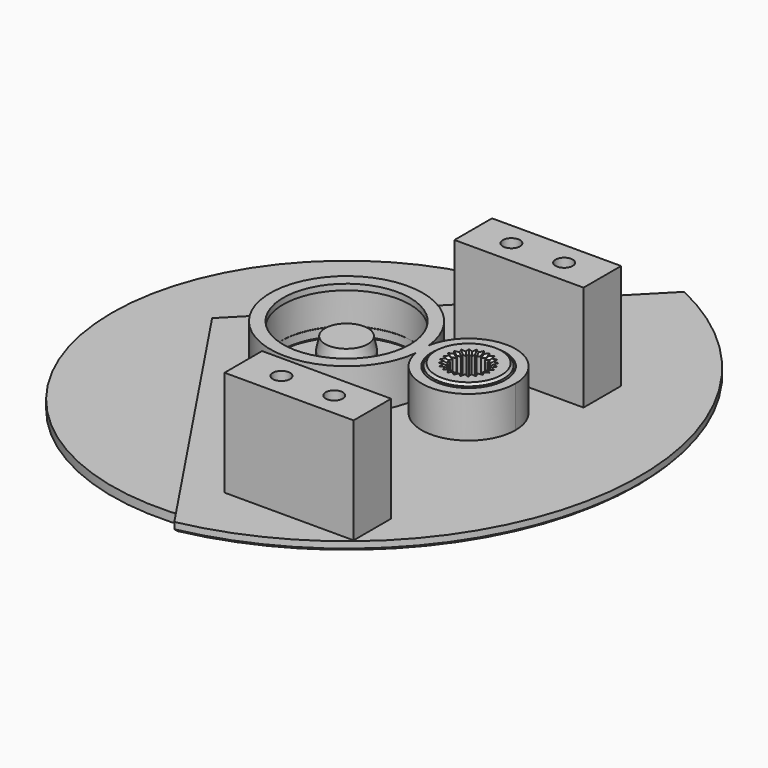
from build123d import *

# Parameters (mm, degrees)
F0_R           = 40
F1_DEPTH       = 1.5
F3_DEPTH       = 3
F4_R           = 4.05
F5_DEPTH       = 6.5
F6_SIZE2       = 2
F6_SIZE        = 0.4
F8_R           = 2
F9_DEPTH       = 2.6
F10_R          = 6
F11_DEPTH      = 9
F12_R          = 11.3
F12_R_2        = 6.2
F13_DEPTH      = 1.5
F14_SIZE       = 0.4
F15_R          = 6.3
F15_R_2        = 11.2
F16_DEPTH      = 7
F17_R          = 11.2
F17_R_2        = 10.8
F18_DEPTH      = 1
F19_C1_SIZE    = 0.4
F19_C2_SIZE    = 0.4
F19_C3_SIZE    = 0.4
F19_C4_SIZE    = 0.4
F19_C5_SIZE    = 0.4
F19_C6_SIZE    = 0.4
F19_C7_SIZE    = 0.4
F19_C8_SIZE    = 0.4
F19_C9_SIZE    = 0.4
F19_C10_SIZE   = 0.4
F19_C11_SIZE   = 0.4
F19_C12_SIZE   = 0.4
F19_C13_SIZE   = 0.4
F19_C14_SIZE   = 0.4
F19_C15_SIZE   = 0.4
F19_C16_SIZE   = 0.4
F19_C17_SIZE   = 0.4
F19_C18_SIZE   = 0.4
F19_C19_SIZE   = 0.4
F19_C20_SIZE   = 0.4
F19_C21_SIZE   = 0.4
F19_C22_SIZE   = 0.4
F19_C23_SIZE   = 0.4
F19_C24_SIZE   = 0.4
F19_C25_SIZE   = 0.4
F19_C26_SIZE   = 0.4
F19_C27_SIZE   = 0.4
F19_C28_SIZE   = 0.4
F19_C29_SIZE   = 0.4
F19_C30_SIZE   = 0.4
F19_C31_SIZE   = 0.4
F19_C32_SIZE   = 0.4
F19_C33_SIZE   = 0.4
F19_C34_SIZE   = 0.4
F19_C35_SIZE   = 0.4
F19_C36_SIZE   = 0.4
F19_C37_SIZE   = 0.4
F19_C38_SIZE   = 0.4
F19_C39_SIZE   = 0.4
F19_C40_SIZE   = 0.4
F19_C41_SIZE   = 0.4
F19_C42_SIZE   = 0.4
F19_C43_SIZE   = 0.4
F19_C44_SIZE   = 0.4
F19_C45_SIZE   = 0.4
F19_C46_SIZE   = 0.4
F19_C47_SIZE   = 0.4
F19_C48_SIZE   = 0.4
F19_C49_SIZE   = 0.4
F19_2_S5_R     = 11.3
F19_2_T6_DEPTH = 18
F21_W          = 22
F21_H          = 8
F21_R          = 1.4665195189
F22_DEPTH      = 18


# Not quite as in the source:
# - a fillet or chamfer that OpenCascade refuses, or shapes differently, is made with other operations: its cross-section is extruded or revolved along the edge and cut away or added


with BuildPart() as f1:
    # F0 (on Top) → F1 (new body)
    with BuildSketch(Plane.XY):
        Circle(F0_R)
    extrude(amount=F1_DEPTH)

    # F2 (on face) → F3 (join)
    with BuildSketch(Plane.XY.offset(1.5)):
        with BuildLine():
            ThreePointArc((6.1294095226, -0.4829629131), (6.3966766701, -0.3043807145), (6.5, 0))
            ThreePointArc((6.5, 0), (6.3966766701, 0.3043807145), (6.1294095226, 0.4829629131))
            ThreePointArc((6.1294095226, 0.4829629131), (5.5, 0), (6.1294095226, -0.4829629131))
        make_face()
        with BuildLine():
            ThreePointArc((6.1294095226, -0.4829629131), (5.5, 0), (6.1294095226, 0.4829629131))
            Line((6.1294095226, 0.4829629131), (4.19755787, 1.0006010033))
            Line((4.19755787, 1.0006010033), (4.1590994684, 1.1144273438))
            Line((4.1590994684, 1.1144273438), (4.1354922509, 1.232233047))
            Line((4.1354922509, 1.232233047), (5.5497058133, 2.6464466094))
            ThreePointArc((5.5497058133, 2.6464466094), (4.7631397208, 2.75), (5.0667429002, 3.4829629131))
            Line((5.0667429002, 3.4829629131), (3.1348912476, 2.9653248229))
            Line((3.1348912476, 2.9653248229), (3.0446721246, 3.0446721246))
            Line((3.0446721246, 3.0446721246), (2.9653248229, 3.1348912476))
            Line((2.9653248229, 3.1348912476), (3.4829629131, 5.0667429002))
            ThreePointArc((3.4829629131, 5.0667429002), (2.75, 4.7631397208), (2.6464466094, 5.5497058133))
            Line((2.6464466094, 5.5497058133), (1.232233047, 4.1354922509))
            Line((1.232233047, 4.1354922509), (1.1144273438, 4.1590994684))
            Line((1.1144273438, 4.1590994684), (1.0006010033, 4.19755787))
            Line((1.0006010033, 4.19755787), (0.4829629131, 6.1294095226))
            ThreePointArc((0.4829629131, 6.1294095226), (0.4957224307, 6.0652630961), (0.5, 6))
            ThreePointArc((0.5, 6), (-0.0652630961, 5.5042775693), (-0.4829629131, 6.1294095226))
            Line((-0.4829629131, 6.1294095226), (-1.0006010033, 4.19755787))
            Line((-1.0006010033, 4.19755787), (-1.1144273438, 4.1590994684))
            Line((-1.1144273438, 4.1590994684), (-1.232233047, 4.1354922509))
            Line((-1.232233047, 4.1354922509), (-2.6464466094, 5.5497058133))
            ThreePointArc((-2.6464466094, 5.5497058133), (-2.5380602337, 5.3874941389), (-2.5, 5.1961524227))
            ThreePointArc((-2.5, 5.1961524227), (-2.9347369039, 4.700429992), (-3.4829629131, 5.0667429002))
            Line((-3.4829629131, 5.0667429002), (-2.9653248229, 3.1348912476))
            Line((-2.9653248229, 3.1348912476), (-3.0446721246, 3.0446721246))
            Line((-3.0446721246, 3.0446721246), (-3.1348912476, 2.9653248229))
            Line((-3.1348912476, 2.9653248229), (-5.0667429002, 3.4829629131))
            ThreePointArc((-5.0667429002, 3.4829629131), (-4.7994757526, 3.3043807145), (-4.6961524227, 3))
            ThreePointArc((-4.6961524227, 3), (-5.0048107065, 2.5380602337), (-5.5497058133, 2.6464466094))
            Line((-5.5497058133, 2.6464466094), (-4.1354922509, 1.232233047))
            Line((-4.1354922509, 1.232233047), (-4.1590994684, 1.1144273438))
            Line((-4.1590994684, 1.1144273438), (-4.19755787, 1.0006010033))
            Line((-4.19755787, 1.0006010033), (-6.1294095226, 0.4829629131))
            ThreePointArc((-6.1294095226, 0.4829629131), (-5.6956192855, 0.3966766701), (-5.5, 0))
            ThreePointArc((-5.5, 0), (-5.6956192855, -0.3966766701), (-6.1294095226, -0.4829629131))
            Line((-6.1294095226, -0.4829629131), (-4.19755787, -1.0006010033))
            Line((-4.19755787, -1.0006010033), (-4.1590994684, -1.1144273438))
            Line((-4.1590994684, -1.1144273438), (-4.1354922509, -1.232233047))
            Line((-4.1354922509, -1.232233047), (-5.5497058133, -2.6464466094))
            ThreePointArc((-5.5497058133, -2.6464466094), (-5.0048107065, -2.5380602337), (-4.6961524227, -3))
            ThreePointArc((-4.6961524227, -3), (-4.7994757526, -3.3043807145), (-5.0667429002, -3.4829629131))
            Line((-5.0667429002, -3.4829629131), (-3.1348912476, -2.9653248229))
            Line((-3.1348912476, -2.9653248229), (-3.0446721246, -3.0446721246))
            Line((-3.0446721246, -3.0446721246), (-2.9653248229, -3.1348912476))
            Line((-2.9653248229, -3.1348912476), (-3.4829629131, -5.0667429002))
            ThreePointArc((-3.4829629131, -5.0667429002), (-2.9347369039, -4.700429992), (-2.5, -5.1961524227))
            ThreePointArc((-2.5, -5.1961524227), (-2.5380602337, -5.3874941389), (-2.6464466094, -5.5497058133))
            Line((-2.6464466094, -5.5497058133), (-1.232233047, -4.1354922509))
            Line((-1.232233047, -4.1354922509), (-1.1144273438, -4.1590994684))
            Line((-1.1144273438, -4.1590994684), (-1.0006010033, -4.19755787))
            Line((-1.0006010033, -4.19755787), (-0.4829629131, -6.1294095226))
            ThreePointArc((-0.4829629131, -6.1294095226), (-0.0652630961, -5.5042775693), (0.5, -6))
            ThreePointArc((0.5, -6), (0.4957224307, -6.0652630961), (0.4829629131, -6.1294095226))
            Line((0.4829629131, -6.1294095226), (1.0006010033, -4.19755787))
            Line((1.0006010033, -4.19755787), (1.1144273438, -4.1590994684))
            Line((1.1144273438, -4.1590994684), (1.232233047, -4.1354922509))
            Line((1.232233047, -4.1354922509), (2.6464466094, -5.5497058133))
            ThreePointArc((2.6464466094, -5.5497058133), (2.75, -4.7631397208), (3.4829629131, -5.0667429002))
            Line((3.4829629131, -5.0667429002), (2.9653248229, -3.1348912476))
            Line((2.9653248229, -3.1348912476), (3.0446721246, -3.0446721246))
            Line((3.0446721246, -3.0446721246), (3.1348912476, -2.9653248229))
            Line((3.1348912476, -2.9653248229), (5.0667429002, -3.4829629131))
            ThreePointArc((5.0667429002, -3.4829629131), (4.7631397208, -2.75), (5.5497058133, -2.6464466094))
            Line((5.5497058133, -2.6464466094), (4.1354922509, -1.232233047))
            Line((4.1354922509, -1.232233047), (4.1590994684, -1.1144273438))
            Line((4.1590994684, -1.1144273438), (4.19755787, -1.0006010033))
            Line((4.19755787, -1.0006010033), (6.1294095226, -0.4829629131))
        make_face()
        with BuildLine():
            ThreePointArc((5.0667429002, 3.4829629131), (4.7631397208, 2.75), (5.5497058133, 2.6464466094))
            ThreePointArc((5.5497058133, 2.6464466094), (5.658092189, 2.8086582838), (5.6961524227, 3))
            ThreePointArc((5.6961524227, 3), (5.5005331372, 3.3966766701), (5.0667429002, 3.4829629131))
        make_face()
        with BuildLine():
            ThreePointArc((5.6961524227, -3), (5.658092189, -2.8086582838), (5.5497058133, -2.6464466094))
            ThreePointArc((5.5497058133, -2.6464466094), (4.7631397208, -2.75), (5.0667429002, -3.4829629131))
            ThreePointArc((5.0667429002, -3.4829629131), (5.5005331372, -3.3966766701), (5.6961524227, -3))
        make_face()
        with BuildLine():
            ThreePointArc((2.6464466094, 5.5497058133), (2.75, 4.7631397208), (3.4829629131, 5.0667429002))
            ThreePointArc((3.4829629131, 5.0667429002), (3.4957224307, 5.1308893266), (3.5, 5.1961524227))
            ThreePointArc((3.5, 5.1961524227), (3.1913417162, 5.658092189), (2.6464466094, 5.5497058133))
        make_face()
        with BuildLine():
            ThreePointArc((3.5, -5.1961524227), (3.4957224307, -5.1308893266), (3.4829629131, -5.0667429002))
            ThreePointArc((3.4829629131, -5.0667429002), (2.75, -4.7631397208), (2.6464466094, -5.5497058133))
            ThreePointArc((2.6464466094, -5.5497058133), (3.1913417162, -5.658092189), (3.5, -5.1961524227))
        make_face()
        with BuildLine():
            ThreePointArc((0.5, 6), (0.4957224307, 6.0652630961), (0.4829629131, 6.1294095226))
            ThreePointArc((0.4829629131, 6.1294095226), (0, 6.5), (-0.4829629131, 6.1294095226))
            ThreePointArc((-0.4829629131, 6.1294095226), (-0.0652630961, 5.5042775693), (0.5, 6))
        make_face()
        with BuildLine():
            ThreePointArc((-0.4829629131, -6.1294095226), (0, -6.5), (0.4829629131, -6.1294095226))
            ThreePointArc((0.4829629131, -6.1294095226), (0.4957224307, -6.0652630961), (0.5, -6))
            ThreePointArc((0.5, -6), (-0.0652630961, -5.5042775693), (-0.4829629131, -6.1294095226))
        make_face()
        with BuildLine():
            ThreePointArc((-2.5, 5.1961524227), (-2.5380602337, 5.3874941389), (-2.6464466094, 5.5497058133))
            ThreePointArc((-2.6464466094, 5.5497058133), (-3.25, 5.6291651246), (-3.4829629131, 5.0667429002))
            ThreePointArc((-3.4829629131, 5.0667429002), (-2.9347369039, 4.700429992), (-2.5, 5.1961524227))
        make_face()
        with BuildLine():
            ThreePointArc((-3.4829629131, -5.0667429002), (-3.25, -5.6291651246), (-2.6464466094, -5.5497058133))
            ThreePointArc((-2.6464466094, -5.5497058133), (-2.5380602337, -5.3874941389), (-2.5, -5.1961524227))
            ThreePointArc((-2.5, -5.1961524227), (-2.9347369039, -4.700429992), (-3.4829629131, -5.0667429002))
        make_face()
        with BuildLine():
            ThreePointArc((-4.6961524227, 3), (-4.7994757526, 3.3043807145), (-5.0667429002, 3.4829629131))
            ThreePointArc((-5.0667429002, 3.4829629131), (-5.6291651246, 3.25), (-5.5497058133, 2.6464466094))
            ThreePointArc((-5.5497058133, 2.6464466094), (-5.0048107065, 2.5380602337), (-4.6961524227, 3))
        make_face()
        with BuildLine():
            ThreePointArc((-5.5497058133, -2.6464466094), (-5.6291651246, -3.25), (-5.0667429002, -3.4829629131))
            ThreePointArc((-5.0667429002, -3.4829629131), (-4.7994757526, -3.3043807145), (-4.6961524227, -3))
            ThreePointArc((-4.6961524227, -3), (-5.0048107065, -2.5380602337), (-5.5497058133, -2.6464466094))
        make_face()
        with BuildLine():
            ThreePointArc((-5.5, 0), (-5.6956192855, 0.3966766701), (-6.1294095226, 0.4829629131))
            ThreePointArc((-6.1294095226, 0.4829629131), (-6.5, 0), (-6.1294095226, -0.4829629131))
            ThreePointArc((-6.1294095226, -0.4829629131), (-5.6956192855, -0.3966766701), (-5.5, 0))
        make_face()
    extrude(amount=F3_DEPTH)

    # F4 (on face) → F5 (join)
    with BuildSketch(Plane.XY.offset(4.5)):
        Circle(F4_R)
    extrude(amount=F5_DEPTH)

    # F6
    f6_edges = [f1.edges().sort_by_distance(p)[0] for p in [
        (-4.05, 0, 11),
    ]]
    f6_side = f1.faces().sort_by_distance((0, 0, 11))[0]
    chamfer(f6_edges, length=F6_SIZE, length2=F6_SIZE2, reference=f6_side)


with BuildPart() as f9:
    # F8 (on offset) → F9 (new body)
    with BuildSketch(Plane.XY.offset(4.75)):
        with BuildLine():
            ThreePointArc((36.005212086, -0.5638155725), (36.2914912266, -0.3441458618), (36.4, 0))
            ThreePointArc((36.4, 0), (36.2914912266, 0.3441458618), (36.005212086, 0.5638155725))
            ThreePointArc((36.005212086, 0.5638155725), (35.2, 0), (36.005212086, -0.5638155725))
        make_face()
        with BuildLine():
            ThreePointArc((36.005212086, -0.5638155725), (35.2, 0), (36.005212086, 0.5638155725))
            Line((36.005212086, 0.5638155725), (34.5956731548, 1.0768457875))
            Line((34.5956731548, 1.0768457875), (34.2894922687, 1.7759253484))
            Line((34.2894922687, 1.7759253484), (34.4043051897, 2.5304297954))
            Line((34.4043051897, 2.5304297954), (35.6330332561, 3.39079445))
            ThreePointArc((35.6330332561, 3.39079445), (34.7093318986, 3.7269942495), (35.34118084, 4.4800024954))
            Line((35.34118084, 4.4800024954), (33.8468887928, 4.6107361095))
            Line((33.8468887928, 4.6107361095), (33.3702056631, 5.2067496675))
            Line((33.3702056631, 5.2067496675), (33.2858263081, 5.9652607695))
            Line((33.2858263081, 5.9652607695), (34.2500077226, 7.1143274342))
            ThreePointArc((34.2500077226, 7.1143274342), (33.2707658145, 7.2), (33.6861921502, 8.0908846518))
            Line((33.6861921502, 8.0908846518), (32.2089805206, 7.8304123853))
            Line((32.2089805206, 7.8304123853), (31.5942803147, 8.2827426013))
            Line((31.5942803147, 8.2827426013), (31.3164589974, 8.9935690802))
            Line((31.3164589974, 8.9935690802), (31.95038639, 10.3530307608))
            ThreePointArc((31.95038639, 10.3530307608), (30.9823376491, 10.1823376491), (31.1530307608, 11.15038639))
            Line((31.1530307608, 11.15038639), (29.7935690802, 10.5164589974))
            Line((29.7935690802, 10.5164589974), (29.0827426013, 10.7942803147))
            Line((29.0827426013, 10.7942803147), (28.6304123853, 11.4089805206))
            Line((28.6304123853, 11.4089805206), (28.8908846518, 12.8861921502))
            ThreePointArc((28.8908846518, 12.8861921502), (28, 12.4707658145), (27.9143274342, 13.4500077226))
            Line((27.9143274342, 13.4500077226), (26.7652607695, 12.4858263081))
            Line((26.7652607695, 12.4858263081), (26.0067496675, 12.5702056631))
            Line((26.0067496675, 12.5702056631), (25.4107361095, 13.0468887928))
            Line((25.4107361095, 13.0468887928), (25.2800024954, 14.54118084))
            ThreePointArc((25.2800024954, 14.54118084), (25.2817146095, 14.5150590268), (25.2822856765, 14.4888873943))
            ThreePointArc((25.2822856765, 14.4888873943), (24.5018621968, 13.9166572239), (24.19079445, 14.8330332561))
            Line((24.19079445, 14.8330332561), (23.3304297954, 13.6043051897))
            Line((23.3304297954, 13.6043051897), (22.5759253484, 13.4894922687))
            Line((22.5759253484, 13.4894922687), (21.8768457875, 13.7956731548))
            Line((21.8768457875, 13.7956731548), (21.3638155725, 15.205212086))
            ThreePointArc((21.3638155725, 15.205212086), (21.3908846518, 15.1041889066), (21.4, 15))
            ThreePointArc((21.4, 15), (20.6958110934, 14.4091153482), (20.2361844275, 15.205212086))
            Line((20.2361844275, 15.205212086), (19.7231542125, 13.7956731548))
            Line((19.7231542125, 13.7956731548), (19.0240746516, 13.4894922687))
            Line((19.0240746516, 13.4894922687), (18.2695702046, 13.6043051897))
            Line((18.2695702046, 13.6043051897), (17.40920555, 14.8330332561))
            ThreePointArc((17.40920555, 14.8330332561), (17.4899444939, 14.669310874), (17.5177143235, 14.4888873943))
            ThreePointArc((17.5177143235, 14.4888873943), (16.891542691, 13.8894584614), (16.3199975046, 14.54118084))
            Line((16.3199975046, 14.54118084), (16.1892638905, 13.0468887928))
            Line((16.1892638905, 13.0468887928), (15.5932503325, 12.5702056631))
            Line((15.5932503325, 12.5702056631), (14.8347392305, 12.4858263081))
            Line((14.8347392305, 12.4858263081), (13.6856725658, 13.4500077226))
            ThreePointArc((13.6856725658, 13.4500077226), (13.8437846722, 13.2439520138), (13.9, 12.9903810568))
            ThreePointArc((13.9, 12.9903810568), (13.3522934456, 12.3926642379), (12.7091153482, 12.8861921502))
            Line((12.7091153482, 12.8861921502), (12.9695876147, 11.4089805206))
            Line((12.9695876147, 11.4089805206), (12.5172573987, 10.7942803147))
            Line((12.5172573987, 10.7942803147), (11.8064309198, 10.5164589974))
            Line((11.8064309198, 10.5164589974), (10.4469692392, 11.15038639))
            ThreePointArc((10.4469692392, 11.15038639), (10.6994331497, 10.9289814828), (10.7933982822, 10.6066017178))
            ThreePointArc((10.7933982822, 10.6066017178), (10.3232620506, 10.0208241135), (9.64961361, 10.3530307608))
            Line((9.64961361, 10.3530307608), (10.2835410026, 8.9935690802))
            Line((10.2835410026, 8.9935690802), (10.0057196853, 8.2827426013))
            Line((10.0057196853, 8.2827426013), (9.3910194794, 7.8304123853))
            Line((9.3910194794, 7.8304123853), (7.9138078498, 8.0908846518))
            ThreePointArc((7.9138078498, 8.0908846518), (8.2692456091, 7.8856725658), (8.4096189432, 7.5))
            ThreePointArc((8.4096189432, 7.5), (8.0148310292, 6.9361844275), (7.3499922774, 7.1143274342))
            Line((7.3499922774, 7.1143274342), (8.3141736919, 5.9652607695))
            Line((8.3141736919, 5.9652607695), (8.2297943369, 5.2067496675))
            Line((8.2297943369, 5.2067496675), (7.7531112072, 4.6107361095))
            Line((7.7531112072, 4.6107361095), (6.25881916, 4.4800024954))
            ThreePointArc((6.25881916, 4.4800024954), (6.7164667302, 4.3246520786), (6.9111126057, 3.8822856765))
            ThreePointArc((6.9111126057, 3.8822856765), (6.5881617736, 3.3500791766), (5.9669667439, 3.39079445))
            Line((5.9669667439, 3.39079445), (7.1956948103, 2.5304297954))
            Line((7.1956948103, 2.5304297954), (7.3105077313, 1.7759253484))
            Line((7.3105077313, 1.7759253484), (7.0043268452, 1.0768457875))
            Line((7.0043268452, 1.0768457875), (5.594787914, 0.5638155725))
            ThreePointArc((5.594787914, 0.5638155725), (6.1441458618, 0.4914912266), (6.4, 0))
            ThreePointArc((6.4, 0), (6.1441458618, -0.4914912266), (5.594787914, -0.5638155725))
            Line((5.594787914, -0.5638155725), (7.0043268452, -1.0768457875))
            Line((7.0043268452, -1.0768457875), (7.3105077313, -1.7759253484))
            Line((7.3105077313, -1.7759253484), (7.1956948103, -2.5304297954))
            Line((7.1956948103, -2.5304297954), (5.9669667439, -3.39079445))
            ThreePointArc((5.9669667439, -3.39079445), (6.5881617736, -3.3500791766), (6.9111126057, -3.8822856765))
            ThreePointArc((6.9111126057, -3.8822856765), (6.7164667302, -4.3246520786), (6.25881916, -4.4800024954))
            Line((6.25881916, -4.4800024954), (7.7531112072, -4.6107361095))
            Line((7.7531112072, -4.6107361095), (8.2297943369, -5.2067496675))
            Line((8.2297943369, -5.2067496675), (8.3141736919, -5.9652607695))
            Line((8.3141736919, -5.9652607695), (7.3499922774, -7.1143274342))
            ThreePointArc((7.3499922774, -7.1143274342), (8.0148310292, -6.9361844275), (8.4096189432, -7.5))
            ThreePointArc((8.4096189432, -7.5), (8.2692456091, -7.8856725658), (7.9138078498, -8.0908846518))
            Line((7.9138078498, -8.0908846518), (9.3910194794, -7.8304123853))
            Line((9.3910194794, -7.8304123853), (10.0057196853, -8.2827426013))
            Line((10.0057196853, -8.2827426013), (10.2835410026, -8.9935690802))
            Line((10.2835410026, -8.9935690802), (9.64961361, -10.3530307608))
            ThreePointArc((9.64961361, -10.3530307608), (10.3232620506, -10.0208241135), (10.7933982822, -10.6066017178))
            ThreePointArc((10.7933982822, -10.6066017178), (10.6994331497, -10.9289814828), (10.4469692392, -11.15038639))
            Line((10.4469692392, -11.15038639), (11.8064309198, -10.5164589974))
            Line((11.8064309198, -10.5164589974), (12.5172573987, -10.7942803147))
            Line((12.5172573987, -10.7942803147), (12.9695876147, -11.4089805206))
            Line((12.9695876147, -11.4089805206), (12.7091153482, -12.8861921502))
            ThreePointArc((12.7091153482, -12.8861921502), (13.3522934456, -12.3926642379), (13.9, -12.9903810568))
            ThreePointArc((13.9, -12.9903810568), (13.8437846722, -13.2439520138), (13.6856725658, -13.4500077226))
            Line((13.6856725658, -13.4500077226), (14.8347392305, -12.4858263081))
            Line((14.8347392305, -12.4858263081), (15.5932503325, -12.5702056631))
            Line((15.5932503325, -12.5702056631), (16.1892638905, -13.0468887928))
            Line((16.1892638905, -13.0468887928), (16.3199975046, -14.54118084))
            ThreePointArc((16.3199975046, -14.54118084), (16.891542691, -13.8894584614), (17.5177143235, -14.4888873943))
            ThreePointArc((17.5177143235, -14.4888873943), (17.4899444939, -14.669310874), (17.40920555, -14.8330332561))
            Line((17.40920555, -14.8330332561), (18.2695702046, -13.6043051897))
            Line((18.2695702046, -13.6043051897), (19.0240746516, -13.4894922687))
            Line((19.0240746516, -13.4894922687), (19.7231542125, -13.7956731548))
            Line((19.7231542125, -13.7956731548), (20.2361844275, -15.205212086))
            ThreePointArc((20.2361844275, -15.205212086), (20.6958110934, -14.4091153482), (21.4, -15))
            ThreePointArc((21.4, -15), (21.3908846518, -15.1041889066), (21.3638155725, -15.205212086))
            Line((21.3638155725, -15.205212086), (21.8768457875, -13.7956731548))
            Line((21.8768457875, -13.7956731548), (22.5759253484, -13.4894922687))
            Line((22.5759253484, -13.4894922687), (23.3304297954, -13.6043051897))
            Line((23.3304297954, -13.6043051897), (24.19079445, -14.8330332561))
            ThreePointArc((24.19079445, -14.8330332561), (24.5018621968, -13.9166572239), (25.2822856765, -14.4888873943))
            ThreePointArc((25.2822856765, -14.4888873943), (25.2817146095, -14.5150590268), (25.2800024954, -14.54118084))
            Line((25.2800024954, -14.54118084), (25.4107361095, -13.0468887928))
            Line((25.4107361095, -13.0468887928), (26.0067496675, -12.5702056631))
            Line((26.0067496675, -12.5702056631), (26.7652607695, -12.4858263081))
            Line((26.7652607695, -12.4858263081), (27.9143274342, -13.4500077226))
            ThreePointArc((27.9143274342, -13.4500077226), (28, -12.4707658145), (28.8908846518, -12.8861921502))
            Line((28.8908846518, -12.8861921502), (28.6304123853, -11.4089805206))
            Line((28.6304123853, -11.4089805206), (29.0827426013, -10.7942803147))
            Line((29.0827426013, -10.7942803147), (29.7935690802, -10.5164589974))
            Line((29.7935690802, -10.5164589974), (31.1530307608, -11.15038639))
            ThreePointArc((31.1530307608, -11.15038639), (30.9823376491, -10.1823376491), (31.95038639, -10.3530307608))
            Line((31.95038639, -10.3530307608), (31.3164589974, -8.9935690802))
            Line((31.3164589974, -8.9935690802), (31.5942803147, -8.2827426013))
            Line((31.5942803147, -8.2827426013), (32.2089805206, -7.8304123853))
            Line((32.2089805206, -7.8304123853), (33.6861921502, -8.0908846518))
            ThreePointArc((33.6861921502, -8.0908846518), (33.2707658145, -7.2), (34.2500077226, -7.1143274342))
            Line((34.2500077226, -7.1143274342), (33.2858263081, -5.9652607695))
            Line((33.2858263081, -5.9652607695), (33.3702056631, -5.2067496675))
            Line((33.3702056631, -5.2067496675), (33.8468887928, -4.6107361095))
            Line((33.8468887928, -4.6107361095), (35.34118084, -4.4800024954))
            ThreePointArc((35.34118084, -4.4800024954), (34.7093318986, -3.7269942495), (35.6330332561, -3.39079445))
            Line((35.6330332561, -3.39079445), (34.4043051897, -2.5304297954))
            Line((34.4043051897, -2.5304297954), (34.2894922687, -1.7759253484))
            Line((34.2894922687, -1.7759253484), (34.5956731548, -1.0768457875))
            Line((34.5956731548, -1.0768457875), (36.005212086, -0.5638155725))
        make_face()
        with Locations((20.8, 0)):
            Circle(F8_R, mode=Mode.SUBTRACT)
        with BuildLine():
            ThreePointArc((35.34118084, 4.4800024954), (34.7093318986, 3.7269942495), (35.6330332561, 3.39079445))
            ThreePointArc((35.6330332561, 3.39079445), (35.8210938942, 3.6052365086), (35.8888873943, 3.8822856765))
            ThreePointArc((35.8888873943, 3.8822856765), (35.7312537964, 4.2876398011), (35.34118084, 4.4800024954))
        make_face()
        with BuildLine():
            ThreePointArc((35.8888873943, -3.8822856765), (35.8210938942, -3.6052365086), (35.6330332561, -3.39079445))
            ThreePointArc((35.6330332561, -3.39079445), (34.7093318986, -3.7269942495), (35.34118084, -4.4800024954))
            ThreePointArc((35.34118084, -4.4800024954), (35.7312537964, -4.2876398011), (35.8888873943, -3.8822856765))
        make_face()
        with BuildLine():
            ThreePointArc((33.6861921502, 8.0908846518), (33.2707658145, 7.2), (34.2500077226, 7.1143274342))
            ThreePointArc((34.2500077226, 7.1143274342), (34.3541966292, 7.294787914), (34.3903810568, 7.5))
            ThreePointArc((34.3903810568, 7.5), (34.1760536226, 7.9596266659), (33.6861921502, 8.0908846518))
        make_face()
        with BuildLine():
            ThreePointArc((34.3903810568, -7.5), (34.3541966292, -7.294787914), (34.2500077226, -7.1143274342))
            ThreePointArc((34.2500077226, -7.1143274342), (33.2707658145, -7.2), (33.6861921502, -8.0908846518))
            ThreePointArc((33.6861921502, -8.0908846518), (34.1760536226, -7.9596266659), (34.3903810568, -7.5))
        make_face()
        with BuildLine():
            ThreePointArc((31.1530307608, 11.15038639), (30.9823376491, 10.1823376491), (31.95038639, 10.3530307608))
            ThreePointArc((31.95038639, 10.3530307608), (31.9923793221, 10.4767379494), (32.0066017178, 10.6066017178))
            ThreePointArc((32.0066017178, 10.6066017178), (31.7289814828, 11.1126365853), (31.1530307608, 11.15038639))
        make_face()
        with BuildLine():
            ThreePointArc((32.0066017178, -10.6066017178), (31.9923793221, -10.4767379494), (31.95038639, -10.3530307608))
            ThreePointArc((31.95038639, -10.3530307608), (30.9823376491, -10.1823376491), (31.1530307608, -11.15038639))
            ThreePointArc((31.1530307608, -11.15038639), (31.7289814828, -11.1126365853), (32.0066017178, -10.6066017178))
        make_face()
        with BuildLine():
            ThreePointArc((27.9143274342, 13.4500077226), (28, 12.4707658145), (28.8908846518, 12.8861921502))
            ThreePointArc((28.8908846518, 12.8861921502), (28.8977168189, 12.9380876111), (28.9, 12.9903810568))
            ThreePointArc((28.9, 12.9903810568), (28.553570957, 13.534165729), (27.9143274342, 13.4500077226))
        make_face()
        with BuildLine():
            ThreePointArc((28.9, -12.9903810568), (28.8977168189, -12.9380876111), (28.8908846518, -12.8861921502))
            ThreePointArc((28.8908846518, -12.8861921502), (28, -12.4707658145), (27.9143274342, -13.4500077226))
            ThreePointArc((27.9143274342, -13.4500077226), (28.553570957, -13.534165729), (28.9, -12.9903810568))
        make_face()
        with BuildLine():
            ThreePointArc((25.2822856765, 14.4888873943), (25.2817146095, 14.5150590268), (25.2800024954, 14.54118084))
            ThreePointArc((25.2800024954, 14.54118084), (24.8375771036, 15.0684428901), (24.19079445, 14.8330332561))
            ThreePointArc((24.19079445, 14.8330332561), (24.5018621968, 13.9166572239), (25.2822856765, 14.4888873943))
        make_face()
        with BuildLine():
            ThreePointArc((24.19079445, -14.8330332561), (24.8375771036, -15.0684428901), (25.2800024954, -14.54118084))
            ThreePointArc((25.2800024954, -14.54118084), (25.2817146095, -14.5150590268), (25.2822856765, -14.4888873943))
            ThreePointArc((25.2822856765, -14.4888873943), (24.5018621968, -13.9166572239), (24.19079445, -14.8330332561))
        make_face()
        with BuildLine():
            ThreePointArc((21.4, 15), (21.3908846518, 15.1041889066), (21.3638155725, 15.205212086))
            ThreePointArc((21.3638155725, 15.205212086), (20.8, 15.6), (20.2361844275, 15.205212086))
            ThreePointArc((20.2361844275, 15.205212086), (20.6958110934, 14.4091153482), (21.4, 15))
        make_face()
        with BuildLine():
            ThreePointArc((20.2361844275, -15.205212086), (20.8, -15.6), (21.3638155725, -15.205212086))
            ThreePointArc((21.3638155725, -15.205212086), (21.3908846518, -15.1041889066), (21.4, -15))
            ThreePointArc((21.4, -15), (20.6958110934, -14.4091153482), (20.2361844275, -15.205212086))
        make_face()
        with BuildLine():
            ThreePointArc((17.5177143235, 14.4888873943), (17.4899444939, 14.669310874), (17.40920555, 14.8330332561))
            ThreePointArc((17.40920555, 14.8330332561), (16.7624228964, 15.0684428901), (16.3199975046, 14.54118084))
            ThreePointArc((16.3199975046, 14.54118084), (16.891542691, 13.8894584614), (17.5177143235, 14.4888873943))
        make_face()
        with BuildLine():
            ThreePointArc((16.3199975046, -14.54118084), (16.7624228964, -15.0684428901), (17.40920555, -14.8330332561))
            ThreePointArc((17.40920555, -14.8330332561), (17.4899444939, -14.669310874), (17.5177143235, -14.4888873943))
            ThreePointArc((17.5177143235, -14.4888873943), (16.891542691, -13.8894584614), (16.3199975046, -14.54118084))
        make_face()
        with BuildLine():
            ThreePointArc((13.9, 12.9903810568), (13.8437846722, 13.2439520138), (13.6856725658, 13.4500077226))
            ThreePointArc((13.6856725658, 13.4500077226), (13, 13.509996299), (12.7091153482, 12.8861921502))
            ThreePointArc((12.7091153482, 12.8861921502), (13.3522934456, 12.3926642379), (13.9, 12.9903810568))
        make_face()
        with BuildLine():
            ThreePointArc((12.7091153482, -12.8861921502), (13, -13.509996299), (13.6856725658, -13.4500077226))
            ThreePointArc((13.6856725658, -13.4500077226), (13.8437846722, -13.2439520138), (13.9, -12.9903810568))
            ThreePointArc((13.9, -12.9903810568), (13.3522934456, -12.3926642379), (12.7091153482, -12.8861921502))
        make_face()
        with BuildLine():
            ThreePointArc((10.7933982822, 10.6066017178), (10.6994331497, 10.9289814828), (10.4469692392, 11.15038639))
            ThreePointArc((10.4469692392, 11.15038639), (9.7691342135, 11.0308657865), (9.64961361, 10.3530307608))
            ThreePointArc((9.64961361, 10.3530307608), (10.3232620506, 10.0208241135), (10.7933982822, 10.6066017178))
        make_face()
        with BuildLine():
            ThreePointArc((9.64961361, -10.3530307608), (9.7691342135, -11.0308657865), (10.4469692392, -11.15038639))
            ThreePointArc((10.4469692392, -11.15038639), (10.6994331497, -10.9289814828), (10.7933982822, -10.6066017178))
            ThreePointArc((10.7933982822, -10.6066017178), (10.3232620506, -10.0208241135), (9.64961361, -10.3530307608))
        make_face()
        with BuildLine():
            ThreePointArc((8.4096189432, 7.5), (8.2692456091, 7.8856725658), (7.9138078498, 8.0908846518))
            ThreePointArc((7.9138078498, 8.0908846518), (7.290003701, 7.8), (7.3499922774, 7.1143274342))
            ThreePointArc((7.3499922774, 7.1143274342), (8.0148310292, 6.9361844275), (8.4096189432, 7.5))
        make_face()
        with BuildLine():
            ThreePointArc((7.3499922774, -7.1143274342), (7.290003701, -7.8), (7.9138078498, -8.0908846518))
            ThreePointArc((7.9138078498, -8.0908846518), (8.2692456091, -7.8856725658), (8.4096189432, -7.5))
            ThreePointArc((8.4096189432, -7.5), (8.0148310292, -6.9361844275), (7.3499922774, -7.1143274342))
        make_face()
        with BuildLine():
            ThreePointArc((6.9111126057, 3.8822856765), (6.7164667302, 4.3246520786), (6.25881916, 4.4800024954))
            ThreePointArc((6.25881916, 4.4800024954), (5.7315571099, 4.0375771036), (5.9669667439, 3.39079445))
            ThreePointArc((5.9669667439, 3.39079445), (6.5881617736, 3.3500791766), (6.9111126057, 3.8822856765))
        make_face()
        with BuildLine():
            ThreePointArc((5.9669667439, -3.39079445), (5.7315571099, -4.0375771036), (6.25881916, -4.4800024954))
            ThreePointArc((6.25881916, -4.4800024954), (6.7164667302, -4.3246520786), (6.9111126057, -3.8822856765))
            ThreePointArc((6.9111126057, -3.8822856765), (6.5881617736, -3.3500791766), (5.9669667439, -3.39079445))
        make_face()
        with BuildLine():
            ThreePointArc((6.4, 0), (6.1441458618, 0.4914912266), (5.594787914, 0.5638155725))
            ThreePointArc((5.594787914, 0.5638155725), (5.2, 0), (5.594787914, -0.5638155725))
            ThreePointArc((5.594787914, -0.5638155725), (6.1441458618, -0.4914912266), (6.4, 0))
        make_face()
    extrude(amount=-F9_DEPTH)

    # F10 (on face) → F11 (join)
    with BuildSketch(Plane.XY.offset(4.75)):
        with Locations((20.8, 0)):
            Circle(F10_R)
        Polygon((24, 0.4346433689), (23.5, 0), (24.0034566258, -0.4083876891), (23.407999731, -0.6988114218), (23.7886029766, -1.2235878009), (23.1382685902, -1.35), (23.3700809733, -1.9554024262), (22.7091883092, -1.9091883092), (22.7764121991, -2.5539596077), (22.15, -2.3382685902), (22.0480541996, -2.9784686624), (21.4988114218, -2.607999731), (21.2346433689, -3.2), (20.8, -2.7), (20.3916123109, -3.2034566258), (20.1011885782, -2.607999731), (19.5764121991, -2.9886029766), (19.45, -2.3382685902), (18.8445975738, -2.5700809733), (18.8908116908, -1.9091883092), (18.2460403923, -1.9764121991), (18.4617314098, -1.35), (17.8215313376, -1.2480541996), (18.192000269, -0.6988114218), (17.6, -0.4346433689), (18.1, 0), (17.5965433742, 0.4083876891), (18.192000269, 0.6988114218), (17.8113970234, 1.2235878009), (18.4617314098, 1.35), (18.2299190267, 1.9554024262), (18.8908116908, 1.9091883092), (18.8235878009, 2.5539596077), (19.45, 2.3382685902), (19.5519458004, 2.9784686624), (20.1011885782, 2.607999731), (20.3653566311, 3.2), (20.8, 2.7), (21.2083876891, 3.2034566258), (21.4988114218, 2.607999731), (22.0235878009, 2.9886029766), (22.15, 2.3382685902), (22.7554024262, 2.5700809733), (22.7091883092, 1.9091883092), (23.3539596077, 1.9764121991), (23.1382685902, 1.35), (23.7784686624, 1.2480541996), (23.407999731, 0.6988114218), align=None, mode=Mode.SUBTRACT)
    extrude(amount=F11_DEPTH)

    # F19: chamfer of 0.4 on 49 edges, made by hand

    # F19_c1
    f19_c1_edges = [f9.edges().sort_by_distance(p)[0] for p in [
        (14.8, 0, 13.75),
    ]]
    chamfer(f19_c1_edges, length=F19_C1_SIZE)

    # F19_c2
    f19_c2_edges = [f9.edges().sort_by_distance(p)[0] for p in [
        (21.7611996114, 2.7983013538, 13.75),
    ]]
    chamfer(f19_c2_edges, length=F19_C2_SIZE)

    # F19_c3
    f19_c3_edges = [f9.edges().sort_by_distance(p)[0] for p in [
        (22.0867939005, 2.6634357834, 13.75),
    ]]
    chamfer(f19_c3_edges, length=F19_C3_SIZE)

    # F19_c4
    f19_c4_edges = [f9.edges().sort_by_distance(p)[0] for p in [
        (22.6423305472, 2.5267850422, 13.75),
    ]]
    chamfer(f19_c4_edges, length=F19_C4_SIZE)

    # F19_c5
    f19_c5_edges = [f9.edges().sort_by_distance(p)[0] for p in [
        (22.7322953677, 2.2396346413, 13.75),
    ]]
    chamfer(f19_c5_edges, length=F19_C5_SIZE)

    # F19_c6
    f19_c6_edges = [f9.edges().sort_by_distance(p)[0] for p in [
        (23.233534748, 1.9638566968, 13.75),
    ]]
    chamfer(f19_c6_edges, length=F19_C6_SIZE)

    # F19_c7
    f19_c7_edges = [f9.edges().sort_by_distance(p)[0] for p in [
        (23.2461140989, 1.6632060995, 13.75),
    ]]
    chamfer(f19_c7_edges, length=F19_C7_SIZE)

    # F19_c8
    f19_c8_edges = [f9.edges().sort_by_distance(p)[0] for p in [
        (23.6588975772, 1.2670947629, 13.75),
    ]]
    chamfer(f19_c8_edges, length=F19_C8_SIZE)

    # F19_c9
    f19_c9_edges = [f9.edges().sort_by_distance(p)[0] for p in [
        (23.5932341967, 0.9734328107, 13.75),
    ]]
    chamfer(f19_c9_edges, length=F19_C9_SIZE)

    # F19_c10
    f19_c10_edges = [f9.edges().sort_by_distance(p)[0] for p in [
        (23.8894312611, 0.4839824148, 13.75),
    ]]
    chamfer(f19_c10_edges, length=F19_C10_SIZE)

    # F19_c11
    f19_c11_edges = [f9.edges().sort_by_distance(p)[0] for p in [
        (23.75, 0.2173216845, 13.75),
    ]]
    chamfer(f19_c11_edges, length=F19_C11_SIZE)

    # F19_c12
    f19_c12_edges = [f9.edges().sort_by_distance(p)[0] for p in [
        (23.9094253101, -0.332112535, 13.75),
    ]]
    chamfer(f19_c12_edges, length=F19_C12_SIZE)

    # F19_c13
    f19_c13_edges = [f9.edges().sort_by_distance(p)[0] for p in [
        (23.7057281784, -0.5535995554, 13.75),
    ]]
    chamfer(f19_c13_edges, length=F19_C13_SIZE)

    # F19_c14
    f19_c14_edges = [f9.edges().sort_by_distance(p)[0] for p in [
        (23.7175171628, -1.1255745643, 13.75),
    ]]
    chamfer(f19_c14_edges, length=F19_C14_SIZE)

    # F19_c15
    f19_c15_edges = [f9.edges().sort_by_distance(p)[0] for p in [
        (23.4634357834, -1.2867939005, 13.75),
    ]]
    chamfer(f19_c15_edges, length=F19_C15_SIZE)

    # F19_c16
    f19_c16_edges = [f9.edges().sort_by_distance(p)[0] for p in [
        (23.3267850422, -1.8423305472, 13.75),
    ]]
    chamfer(f19_c16_edges, length=F19_C16_SIZE)

    # F19_c17
    f19_c17_edges = [f9.edges().sort_by_distance(p)[0] for p in [
        (23.0396346413, -1.9322953677, 13.75),
    ]]
    chamfer(f19_c17_edges, length=F19_C17_SIZE)

    # F19_c18
    f19_c18_edges = [f9.edges().sort_by_distance(p)[0] for p in [
        (22.7638566968, -2.433534748, 13.75),
    ]]
    chamfer(f19_c18_edges, length=F19_C18_SIZE)

    # F19_c19
    f19_c19_edges = [f9.edges().sort_by_distance(p)[0] for p in [
        (22.4632060995, -2.4461140989, 13.75),
    ]]
    chamfer(f19_c19_edges, length=F19_C19_SIZE)

    # F19_c20
    f19_c20_edges = [f9.edges().sort_by_distance(p)[0] for p in [
        (22.0670947629, -2.8588975772, 13.75),
    ]]
    chamfer(f19_c20_edges, length=F19_C20_SIZE)

    # F19_c21
    f19_c21_edges = [f9.edges().sort_by_distance(p)[0] for p in [
        (21.7734328107, -2.7932341967, 13.75),
    ]]
    chamfer(f19_c21_edges, length=F19_C21_SIZE)

    # F19_c22
    f19_c22_edges = [f9.edges().sort_by_distance(p)[0] for p in [
        (21.2839824148, -3.0894312611, 13.75),
    ]]
    chamfer(f19_c22_edges, length=F19_C22_SIZE)

    # F19_c23
    f19_c23_edges = [f9.edges().sort_by_distance(p)[0] for p in [
        (21.0173216845, -2.95, 13.75),
    ]]
    chamfer(f19_c23_edges, length=F19_C23_SIZE)

    # F19_c24
    f19_c24_edges = [f9.edges().sort_by_distance(p)[0] for p in [
        (20.467887465, -3.1094253101, 13.75),
    ]]
    chamfer(f19_c24_edges, length=F19_C24_SIZE)

    # F19_c25
    f19_c25_edges = [f9.edges().sort_by_distance(p)[0] for p in [
        (20.2464004446, -2.9057281784, 13.75),
    ]]
    chamfer(f19_c25_edges, length=F19_C25_SIZE)

    # F19_c26
    f19_c26_edges = [f9.edges().sort_by_distance(p)[0] for p in [
        (19.6744254357, -2.9175171628, 13.75),
    ]]
    chamfer(f19_c26_edges, length=F19_C26_SIZE)

    # F19_c27
    f19_c27_edges = [f9.edges().sort_by_distance(p)[0] for p in [
        (19.5132060995, -2.6634357834, 13.75),
    ]]
    chamfer(f19_c27_edges, length=F19_C27_SIZE)

    # F19_c28
    f19_c28_edges = [f9.edges().sort_by_distance(p)[0] for p in [
        (18.9576694528, -2.5267850422, 13.75),
    ]]
    chamfer(f19_c28_edges, length=F19_C28_SIZE)

    # F19_c29
    f19_c29_edges = [f9.edges().sort_by_distance(p)[0] for p in [
        (18.8677046323, -2.2396346413, 13.75),
    ]]
    chamfer(f19_c29_edges, length=F19_C29_SIZE)

    # F19_c30
    f19_c30_edges = [f9.edges().sort_by_distance(p)[0] for p in [
        (18.366465252, -1.9638566968, 13.75),
    ]]
    chamfer(f19_c30_edges, length=F19_C30_SIZE)

    # F19_c31
    f19_c31_edges = [f9.edges().sort_by_distance(p)[0] for p in [
        (18.3538859011, -1.6632060995, 13.75),
    ]]
    chamfer(f19_c31_edges, length=F19_C31_SIZE)

    # F19_c32
    f19_c32_edges = [f9.edges().sort_by_distance(p)[0] for p in [
        (17.9411024228, -1.2670947629, 13.75),
    ]]
    chamfer(f19_c32_edges, length=F19_C32_SIZE)

    # F19_c33
    f19_c33_edges = [f9.edges().sort_by_distance(p)[0] for p in [
        (18.0067658033, -0.9734328107, 13.75),
    ]]
    chamfer(f19_c33_edges, length=F19_C33_SIZE)

    # F19_c34
    f19_c34_edges = [f9.edges().sort_by_distance(p)[0] for p in [
        (17.7105687389, -0.4839824148, 13.75),
    ]]
    chamfer(f19_c34_edges, length=F19_C34_SIZE)

    # F19_c35
    f19_c35_edges = [f9.edges().sort_by_distance(p)[0] for p in [
        (17.85, -0.2173216845, 13.75),
    ]]
    chamfer(f19_c35_edges, length=F19_C35_SIZE)

    # F19_c36
    f19_c36_edges = [f9.edges().sort_by_distance(p)[0] for p in [
        (17.6905746899, 0.332112535, 13.75),
    ]]
    chamfer(f19_c36_edges, length=F19_C36_SIZE)

    # F19_c37
    f19_c37_edges = [f9.edges().sort_by_distance(p)[0] for p in [
        (17.8942718216, 0.5535995554, 13.75),
    ]]
    chamfer(f19_c37_edges, length=F19_C37_SIZE)

    # F19_c38
    f19_c38_edges = [f9.edges().sort_by_distance(p)[0] for p in [
        (17.8824828372, 1.1255745643, 13.75),
    ]]
    chamfer(f19_c38_edges, length=F19_C38_SIZE)

    # F19_c39
    f19_c39_edges = [f9.edges().sort_by_distance(p)[0] for p in [
        (18.1365642166, 1.2867939005, 13.75),
    ]]
    chamfer(f19_c39_edges, length=F19_C39_SIZE)

    # F19_c40
    f19_c40_edges = [f9.edges().sort_by_distance(p)[0] for p in [
        (18.2732149578, 1.8423305472, 13.75),
    ]]
    chamfer(f19_c40_edges, length=F19_C40_SIZE)

    # F19_c41
    f19_c41_edges = [f9.edges().sort_by_distance(p)[0] for p in [
        (18.5603653587, 1.9322953677, 13.75),
    ]]
    chamfer(f19_c41_edges, length=F19_C41_SIZE)

    # F19_c42
    f19_c42_edges = [f9.edges().sort_by_distance(p)[0] for p in [
        (18.8361433032, 2.433534748, 13.75),
    ]]
    chamfer(f19_c42_edges, length=F19_C42_SIZE)

    # F19_c43
    f19_c43_edges = [f9.edges().sort_by_distance(p)[0] for p in [
        (19.1367939005, 2.4461140989, 13.75),
    ]]
    chamfer(f19_c43_edges, length=F19_C43_SIZE)

    # F19_c44
    f19_c44_edges = [f9.edges().sort_by_distance(p)[0] for p in [
        (19.5329052371, 2.8588975772, 13.75),
    ]]
    chamfer(f19_c44_edges, length=F19_C44_SIZE)

    # F19_c45
    f19_c45_edges = [f9.edges().sort_by_distance(p)[0] for p in [
        (19.8265671893, 2.7932341967, 13.75),
    ]]
    chamfer(f19_c45_edges, length=F19_C45_SIZE)

    # F19_c46
    f19_c46_edges = [f9.edges().sort_by_distance(p)[0] for p in [
        (20.3160175852, 3.0894312611, 13.75),
    ]]
    chamfer(f19_c46_edges, length=F19_C46_SIZE)

    # F19_c47
    f19_c47_edges = [f9.edges().sort_by_distance(p)[0] for p in [
        (20.5826783155, 2.95, 13.75),
    ]]
    chamfer(f19_c47_edges, length=F19_C47_SIZE)

    # F19_c48
    f19_c48_edges = [f9.edges().sort_by_distance(p)[0] for p in [
        (21.132112535, 3.1094253101, 13.75),
    ]]
    chamfer(f19_c48_edges, length=F19_C48_SIZE)

    # F19_c49
    f19_c49_edges = [f9.edges().sort_by_distance(p)[0] for p in [
        (21.264585885, 3.0882332489, 13.75),
    ]]
    chamfer(f19_c49_edges, length=F19_C49_SIZE)


with BuildPart() as f13:
    # F12 (on offset) → F13 (new body)
    with BuildSketch(Plane.XY.offset(4.75)):
        with BuildLine():
            Line((-22.9172576219, 0), (9.8503120175, -49.0201117212))
            ThreePointArc((9.8503120175, -49.0201117212), (49.6275228275, -6.0917138808), (21.4135615461, 45.1825119035))
            Line((21.4135615461, 45.1825119035), (-22.9172576219, 0))
        make_face()
        Circle(F12_R, mode=Mode.SUBTRACT)
        with Locations((20.8, 0)):
            Circle(F12_R_2, mode=Mode.SUBTRACT)
    extrude(amount=F13_DEPTH)

    # F14
    f14_edges = [f13.edges().sort_by_distance(p)[0] for p in [
        (-0.751848, 22.591256, 4.75),
        (-6.533473, -24.510056, 4.75),
        (49.627523, -6.091714, 4.75),
        (-11.3, 0, 4.75),
        (14.6, 0, 4.75),
    ]]
    chamfer(f14_edges, length=F14_SIZE)

    # F15 (on face) → F16 (join)
    with BuildSketch(Plane.XY.offset(6.25)):
        with BuildLine():
            ThreePointArc((12.9240384615, -1.4032925015), (12.9809957245, -0.7026734661), (13, 0))
            ThreePointArc((13, 0), (12.9809957245, 0.7026734661), (12.9240384615, 1.4032925015))
            ThreePointArc((12.9240384615, 1.4032925015), (12.8, 0), (12.9240384615, -1.4032925015))
        make_face()
        with BuildLine():
            ThreePointArc((12.9240384615, 1.4032925015), (12.9809957245, 0.7026734661), (13, 0))
            ThreePointArc((13, 0), (12.9809957245, -0.7026734661), (12.9240384615, -1.4032925015))
            ThreePointArc((12.9240384615, -1.4032925015), (21.5043818894, -7.9689300508), (28.8, 0))
            ThreePointArc((28.8, 0), (21.5043818894, 7.9689300508), (12.9240384615, 1.4032925015))
        make_face()
        with Locations((20.8, 0)):
            Circle(F15_R, mode=Mode.SUBTRACT)
        with BuildLine():
            ThreePointArc((12.9240384615, -1.4032925015), (12.8, 0), (12.9240384615, 1.4032925015))
            ThreePointArc((12.9240384615, 1.4032925015), (-13, 0), (12.9240384615, -1.4032925015))
        make_face()
        Circle(F15_R_2, mode=Mode.SUBTRACT)
    extrude(amount=F16_DEPTH)

    # F17 (on face) → F18 (join)
    with BuildSketch(Plane.XY.offset(13.25)):
        Circle(F17_R)
        Circle(F17_R_2, mode=Mode.SUBTRACT)
    extrude(amount=-F18_DEPTH)

    # F19#2: chamfer of 0.4 on 1 edges, made by hand


with BuildPart() as f19_2_tool2:
    # F19_2_s3 → F19_2_t4 (revolve)
    with BuildSketch(Plane.XZ):
        Polygon((11.6, 6.25), (11.2, 6.65), (11.2, 6.25), align=None)
    revolve(axis=Axis((0, 0, 6.25), (0, 0, 1)))

    # F19_2_s5 → F19_2_t6 (intersect, symmetric)
    with BuildSketch(Plane.XY.offset(6.5)):
        Circle(F19_2_S5_R)
    extrude(amount=F19_2_T6_DEPTH, both=True, mode=Mode.INTERSECT)


with BuildPart() as f13_1:
    add(f13.part)

    # F19_2_t1: cut F19_2_tool2
    add(f19_2_tool2.part, mode=Mode.SUBTRACT)

    # F21 (on face) → F22 (join)
    with BuildSketch(Plane.XY.offset(6.25)):
        with Locations((20.8, 14.75)):
            Rectangle(F21_W, F21_H)
        with Locations((16.3, 14.75)):
            Circle(F21_R, mode=Mode.SUBTRACT)
        with Locations((25.3, 14.75)):
            Circle(F21_R, mode=Mode.SUBTRACT)
        with Locations((20.8, -34.25)):
            Rectangle(F21_W, F21_H)
        with Locations((16.3, -34.25)):
            Circle(F21_R, mode=Mode.SUBTRACT)
        with Locations((25.3, -34.25)):
            Circle(F21_R, mode=Mode.SUBTRACT)
    extrude(amount=F22_DEPTH)


solid = Compound([f1.part, f9.part, f13_1.part])
